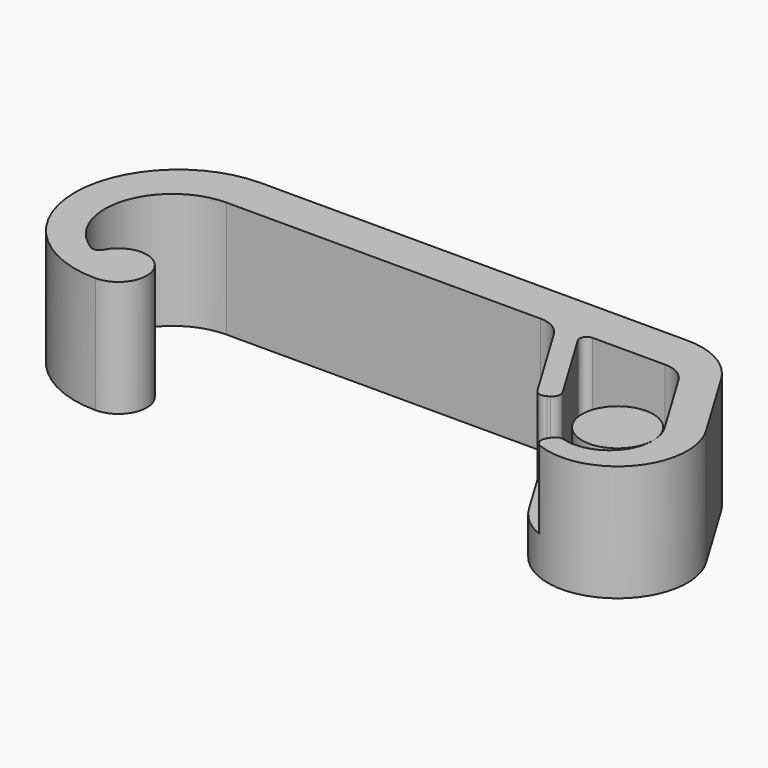
from build123d import *

# Parameters (mm, degrees)
F1_DEPTH       = 8.2
F2_DEPTH       = 1
F4_DEPTH       = 5.5
F16_DEPTH      = 5.5
F5_R           = 2
F17_R          = 0.5
F18_R          = 2
F19_R          = 5
F20_R          = 0.5
F6_R           = 0.6
F8_DEPTH       = 1.5
F9_T4_ANGLE    = 11.9082557293
F10_T4_ANGLE   = 11.9082557293
F11_R          = 2.5
F12_DEPTH      = 4
F13_W          = 47.1088511404
F13_H          = 11.3580938778
F14_DEPTH      = 9.9662867391
F14_DEPTH_BACK = 5.6739057342


# Not quite as in the source:
# - a fillet or chamfer that OpenCascade refuses, or shapes differently, is made with other operations: its cross-section is extruded or revolved along the edge and cut away or added


with BuildPart() as f1:
    # F0 (on Top) → F1 (new body, symmetric)
    with BuildSketch(Plane.XY):
        with BuildLine():
            Line((-7.1751643711, 9.4652866391), (-39.9751643711, 9.4652866391))
            ThreePointArc((-39.9751643711, 9.4652866391), (-47.2251643711, 2.2152866391), (-39.9751643711, -5.0347133609))
            ThreePointArc((-39.9751643711, -5.0347133609), (-38.4191911607, -1.778151636), (-41.9303407523, -2.6136607293))
            ThreePointArc((-41.9303407523, -2.6136607293), (-44.6187082764, 2.7152866391), (-39.9751643711, 6.4652866391))
            Line((-39.9751643711, 6.4652866391), (-16.8055898067, 6.4652866391))
            Line((-16.8055898067, 6.4652866391), (-10.9400612438, -3.2965922013))
            ThreePointArc((-10.9400612438, -3.2965922013), (-4.2162549033, -4.9730254077), (-2.5398216969, 1.7507809328))
            Line((-2.5398216969, 1.7507809328), (-7.1751643711, 9.4652866391))
        make_face()
        with BuildLine():
            Line((-15.1723030506, 6.4652866391), (-8.0558393276, 6.4652866391))
            Line((-8.0558393276, 6.4652866391), (-4.5113064885, 0.5661933605))
            ThreePointArc((-4.5113064885, 0.5661933605), (-5.5548006272, -3.6190330351), (-9.7400270228, -2.5755388964))
            Line((-9.7400270228, -2.5755388964), (-15.1723030506, 6.4652866391))
        make_face(mode=Mode.SUBTRACT)
    extrude(amount=F1_DEPTH, both=True)

    # F0 (on Top) → F2 (join, symmetric)
    with BuildSketch(Plane.XY):
        with BuildLine():
            Line((-4.5113064885, 0.5661933605), (-8.0558393276, 6.4652866391))
            Line((-8.0558393276, 6.4652866391), (-15.1723030506, 6.4652866391))
            Line((-15.1723030506, 6.4652866391), (-9.7400270228, -2.5755388964))
            ThreePointArc((-9.7400270228, -2.5755388964), (-5.5548006272, -3.6190330351), (-4.5113064885, 0.5661933605))
        make_face()
    extrude(amount=F2_DEPTH, both=True)

    # F3 (on face) → F4 (cut)
    with BuildSketch(Plane.XY.offset(8.2)):
        Polygon((-10.0407510024, -6.6778307382), (-6.7399414704, -0.7729056342), (-8.2276463966, 1.7030511502), (-13.2597389706, -1.3205351088), align=None)
    extrude(amount=-F4_DEPTH, mode=Mode.SUBTRACT)

    # F15 (on face) → F16 (cut)
    with BuildSketch(Plane(origin=(0, 0, -8.2), x_dir=(1, 0, 0), z_dir=(0, 0, -1))):
        with BuildLine():
            Line((-12.42776617, 0.8206354168), (-11.227731949, 0.099582112))
            Line((-11.227731949, 0.099582112), (-9.7400270228, 2.5755388964))
            ThreePointArc((-9.7400270228, 2.5755388964), (-9.166526222, 3.2712544759), (-8.4146795695, 3.7688988741))
            Line((-8.4146795695, 3.7688988741), (-9.130817206, 5.0500206919))
            ThreePointArc((-9.130817206, 5.0500206919), (-10.1500636556, 4.2915796291), (-10.9400612438, 3.2965922013))
            Line((-10.9400612438, 3.2965922013), (-12.42776617, 0.8206354168))
        make_face()
    extrude(amount=-F16_DEPTH, mode=Mode.SUBTRACT)

    # F5
    f5_edges = [f1.edges().sort_by_distance(p)[0] for p in [
        (-16.80559, 6.465287, 0),
    ]]
    fillet(f5_edges, radius=F5_R)

    # F17
    f17_edges = [f1.edges().sort_by_distance(p)[0] for p in [
        (-15.172303, 6.465287, -4.6),
        (-15.172303, 6.465287, 4.6),
    ]]
    fillet(f17_edges, radius=F17_R)

    # F18
    f18_edges = [f1.edges().sort_by_distance(p)[0] for p in [
        (-8.055839, 6.465287, -4.6),
        (-8.055839, 6.465287, 4.6),
    ]]
    fillet(f18_edges, radius=F18_R)

    # F19
    f19_edges = [f1.edges().sort_by_distance(p)[0] for p in [
        (-7.175164, 9.465287, 0),
    ]]
    fillet(f19_edges, radius=F19_R)

    # F20
    f20_edges = [f1.edges().sort_by_distance(p)[0] for p in [
        (-41.930341, -2.613661, 0),
    ]]
    fillet(f20_edges, radius=F20_R)

    # F6
    f6_edges = [f1.edges().sort_by_distance(p)[0] for p in [
        (-12.427766, -0.820635, 5.45),
        (-11.227732, -0.099582, 5.45),
        (-8.41468, -3.768899, 5.45),
        (-9.130817, -5.050021, 5.45),
        (-9.130817, -5.050021, -5.45),
        (-8.41468, -3.768899, -5.45),
        (-12.427766, -0.820635, -5.45),
        (-11.227732, -0.099582, -5.45),
    ]]
    fillet(f6_edges, radius=F6_R)

    # F7 (on Top) → F8 (join, symmetric)
    with BuildSketch(Plane.XY):
        with BuildLine():
            ThreePointArc((-12.9599444568, 9.4652866391), (-25.4599444568, 9.9652866391), (-37.9599444568, 9.4652866391))
            Line((-37.9599444568, 9.4652866391), (-12.9599444568, 9.4652866391))
        make_face()
    extrude(amount=F8_DEPTH, both=True)

    # F9: fillet of radius 1.5 on 1 edges, made by hand


with BuildPart() as f9_tool2:
    # F9_s3 → F9_t4 (revolve)
    with BuildSketch(Plane(origin=(-10.0676204433, 1.0500008536, 0), x_dir=(0, 0, 1), z_dir=(0.9946052642, -0.1037321959, 0))):
        with BuildLine():
            ThreePointArc((1.5, -6.6147867599), (1.0606601718, -7.6754469317), (0, -8.1147867599))
            Line((0, -8.1147867599), (1.5, -8.1147867599))
            Line((1.5, -8.1147867599), (1.5, -6.6147867599))
        make_face()
    revolve(axis=Axis((-25.4599444568, -146.5347133609, 1.5), (0, 0, 1)), revolution_arc=F9_T4_ANGLE)

    split(bisect_by=Plane.XZ.offset(-9.4652866391), keep=Keep.BOTTOM)


with BuildPart() as f1_1:
    add(f1.part)

    # F9_t1: cut F9_tool2
    add(f9_tool2.part, mode=Mode.SUBTRACT)

    # F10: fillet of radius 1.5 on 1 edges, made by hand


with BuildPart() as f10_tool2:
    # F10_s3 → F10_t4 (revolve)
    with BuildSketch(Plane(origin=(-10.0676204433, 1.0500008536, 0), x_dir=(0, 0, 1), z_dir=(0.9946052642, -0.1037321959, 0))):
        with BuildLine():
            ThreePointArc((0, -8.1147867599), (-1.0606601718, -7.6754469317), (-1.5, -6.6147867599))
            Line((-1.5, -6.6147867599), (-1.5, -8.1147867599))
            Line((-1.5, -8.1147867599), (0, -8.1147867599))
        make_face()
    revolve(axis=Axis((-25.4599444568, -146.5347133609, -1.5), (0, 0, 1)), revolution_arc=F10_T4_ANGLE)

    split(bisect_by=Plane.XZ.offset(-9.4652866391), keep=Keep.BOTTOM)


with BuildPart() as f1_2:
    add(f1_1.part)

    # F10_t1: cut F10_tool2
    add(f10_tool2.part, mode=Mode.SUBTRACT)

    # F13 (on Front) → F14 (cut, two sides)
    with BuildSketch(Plane.XZ) as f14_sk:
        with Locations((-24.7634426923, -5.6371351529)):
            Rectangle(F13_W, F13_H)
    extrude(amount=-F14_DEPTH, mode=Mode.SUBTRACT)
    extrude(f14_sk.sketch, amount=F14_DEPTH_BACK, mode=Mode.SUBTRACT)


with BuildPart() as f12:
    # F11 (on face) → F12 (new body)
    with BuildSketch(Plane.XY.offset(8.2)):
        with Locations((-6.5767139877, -0.9707484622)):
            Circle(F11_R)
    extrude(amount=-F12_DEPTH)


solid = Compound([f1_2.part, f12.part])
